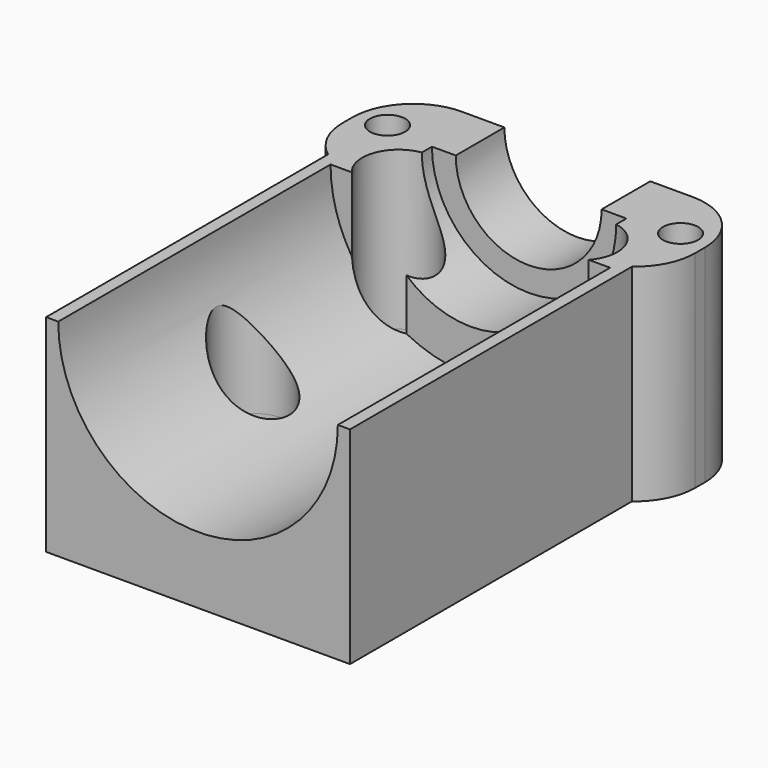
from build123d import *

# Parameters (mm, degrees)
F0_W           = 25
F0_H           = 30
F1_DEPTH       = 4
F2_W           = 25
F2_H           = 11
F3_DEPTH       = 13
F4_R           = 1.675
F5_DEPTH       = 25
F5_DEPTH_BACK  = 25
F7_DEPTH       = 6
F8_R           = 8
F9_DEPTH       = 6
F4_R_2         = 3
F10_DEPTH      = 2
F10_DEPTH_BACK = 25
F12_DEPTH      = 2
F13_W          = 11
F13_H          = 17
F14_DEPTH      = 2
F15_R          = 1.45
F16_DEPTH      = 25
F17_T1_DEPTH   = 42
F17_T6_DEPTH   = 41.9721204096
F17_T11_DEPTH  = 41.9721204096
F18_DEPTH      = 9
F19_DEPTH      = 13
F21_DEPTH      = 28


# Not quite as in the source:
# - a fillet or chamfer that OpenCascade refuses, or shapes differently, is made with other operations: its cross-section is extruded or revolved along the edge and cut away or added
# - a feature names something its author has since deleted; it is built from what else it names


with BuildPart() as f1:
    # F0 (on Top) → F1 (new body)
    with BuildSketch(Plane.XY):
        with Locations((12.5, 15)):
            Rectangle(F0_W, F0_H)
    extrude(amount=F1_DEPTH)

    # F2 (on face) → F3 (join)
    with BuildSketch(Plane.XY.offset(4)):
        with Locations((12.5, 24.5)):
            Rectangle(F2_W, F2_H)
    extrude(amount=F3_DEPTH)

    # F4 (on face) → F5 (cut, two sides)
    with BuildSketch(Plane.XY.offset(4)) as f5_sk:
        with Locations((5, 21)):
            Circle(F4_R)
        with Locations((20, 21)):
            Circle(F4_R)
        with Locations((20, 6)):
            Circle(F4_R)
        with Locations((5, 6)):
            Circle(F4_R)
    extrude(amount=-F5_DEPTH, mode=Mode.SUBTRACT)
    extrude(f5_sk.sketch, amount=F5_DEPTH_BACK, mode=Mode.SUBTRACT)

    # F6 (on face) → F7 (cut)
    with BuildSketch(Plane(origin=(0, 30, 0), x_dir=(-1, 0, 0), z_dir=(0, 1, 0))):
        with BuildLine():
            ThreePointArc((-18.5, 17), (-12.5, 11), (-6.5, 17))
            Line((-6.5, 17), (-18.5, 17))
        make_face()
    extrude(amount=-F7_DEPTH, mode=Mode.SUBTRACT)

    # F8 (on face) → F9 (cut)
    with BuildSketch(Plane.XZ.offset(-19)):
        with Locations((12.5394891948, 17)):
            Circle(F8_R)
    extrude(amount=-F9_DEPTH, mode=Mode.SUBTRACT)

    # F4 (on face) → F10 (cut, two sides)
    with BuildSketch(Plane.XY.offset(4)) as f10_sk:
        with BuildLine():
            ThreePointArc((7.2360679775, 19), (7.8025170769, 19.9295337307), (8, 21))
            ThreePointArc((8, 21), (3.9295337307, 23.8025170769), (2.7639320225, 19))
            Line((2.7639320225, 19), (7.2360679775, 19))
        make_face()
        with Locations((5, 21)):
            Circle(F4_R, mode=Mode.SUBTRACT)
        with BuildLine():
            ThreePointArc((23, 21), (18.9295337307, 23.8025170769), (17.7639320225, 19))
            Line((17.7639320225, 19), (22.2360679775, 19))
            ThreePointArc((22.2360679775, 19), (22.8025170769, 19.9295337307), (23, 21))
        make_face()
        with Locations((20, 21)):
            Circle(F4_R, mode=Mode.SUBTRACT)
        with Locations((20, 6)):
            Circle(F4_R_2)
        with Locations((20, 6)):
            Circle(F4_R, mode=Mode.SUBTRACT)
        with Locations((5, 6)):
            Circle(F4_R_2)
        with Locations((5, 6)):
            Circle(F4_R, mode=Mode.SUBTRACT)
        with BuildLine():
            Line((22.2360679775, 19), (17.7639320225, 19))
            ThreePointArc((17.7639320225, 19), (20, 18), (22.2360679775, 19))
        make_face()
        with BuildLine():
            Line((7.2360679775, 19), (2.7639320225, 19))
            ThreePointArc((2.7639320225, 19), (5, 18), (7.2360679775, 19))
        make_face()
    extrude(amount=-F10_DEPTH, mode=Mode.SUBTRACT)
    extrude(f10_sk.sketch, amount=F10_DEPTH_BACK, mode=Mode.SUBTRACT)

    # F11 (on face) → F12 (join)
    with BuildSketch(Plane(origin=(0, 0, 0), x_dir=(0, -1, 0), z_dir=(-1, 0, 0))):
        Polygon((-30, 17), (-30, 0), (-19, 0), (-19, 4), (-19, 17), align=None)
    extrude(amount=F12_DEPTH)

    # F13 (on face) → F14 (join)
    with BuildSketch(Plane.YZ.offset(25)):
        with Locations((24.5, 8.5)):
            Rectangle(F13_W, F13_H)
    extrude(amount=F14_DEPTH)

    # F15 (on face) → F16 (cut)
    with BuildSketch(Plane.XY.offset(17)):
        with Locations((0.45, 25.55)):
            Circle(F15_R)
        with Locations((24.55, 25.55)):
            Circle(F15_R)
    extrude(amount=-F16_DEPTH, mode=Mode.SUBTRACT)

    # F17: fillet of radius 5 on 4 edges, made by hand

    # F17_s2 → F17_t1 (cut)
    with BuildSketch(Plane.XY.offset(-12.5)):
        with BuildLine():
            ThreePointArc((-2, 25), (-0.5355339059, 28.5355339059), (3, 30))
            Line((3, 30), (-2, 30))
            Line((-2, 30), (-2, 25))
        make_face()
        with BuildLine():
            ThreePointArc((22, 30), (25.5355339059, 28.5355339059), (27, 25))
            Line((27, 25), (27, 30))
            Line((27, 30), (22, 30))
        make_face()
    extrude(amount=F17_T1_DEPTH, mode=Mode.SUBTRACT)


with BuildPart() as f17_tool4:
    # F17_s5 → F17_t6 (new body)
    with BuildSketch(Plane.XY.offset(29.4860602048)):
        with BuildLine():
            ThreePointArc((2.7639320225, 19), (-0.6180339887, 20.5433619184), (-2, 23.9944240819))
            Line((-2, 23.9944240819), (-2, 19))
            Line((-2, 19), (2.7639320225, 19))
        make_face()
    extrude(amount=-F17_T6_DEPTH)

    split(bisect_by=Plane.YZ, keep=Keep.BOTTOM)


with BuildPart() as f1_1:
    add(f1.part)

    # F17_t3: cut F17_tool4
    add(f17_tool4.part, mode=Mode.SUBTRACT)


with BuildPart() as f17_tool9:
    # F17_s10 → F17_t11 (new body)
    with BuildSketch(Plane.XY.offset(29.4860602048)):
        with BuildLine():
            ThreePointArc((22.2360679775, 19), (25.6180339887, 20.5433619184), (27, 23.9944240819))
            Line((27, 23.9944240819), (27, 19))
            Line((27, 19), (22.2360679775, 19))
        make_face()
    extrude(amount=-F17_T11_DEPTH)

    split(bisect_by=Plane.YZ.offset(25), keep=Keep.TOP)


with BuildPart() as f1_2:
    add(f1_1.part)

    # F17_t8: cut F17_tool9
    add(f17_tool9.part, mode=Mode.SUBTRACT)

    # F18 (add): a face of the model
    f18_faces = [f1_2.faces().sort_by_distance(p)[0] for p in [
        (12.5, 0, 2),
    ]]
    extrude(f18_faces, amount=F18_DEPTH)

    # F19 (add): a face of the model
    f19_faces = [f1_2.faces().sort_by_distance(p)[0] for p in [
        (12.5, 4.7791140559, 4),
    ]]
    extrude(f19_faces, amount=F19_DEPTH)

    # F20 (on face) → F21 (cut, through all)
    with BuildSketch(Plane.XZ.offset(9)):
        with BuildLine():
            ThreePointArc((1, 17), (12.5, 5.5), (24, 17))
            Line((24, 17), (1, 17))
        make_face()
    extrude(amount=-F21_DEPTH, mode=Mode.SUBTRACT)


solid = f1_2.part
